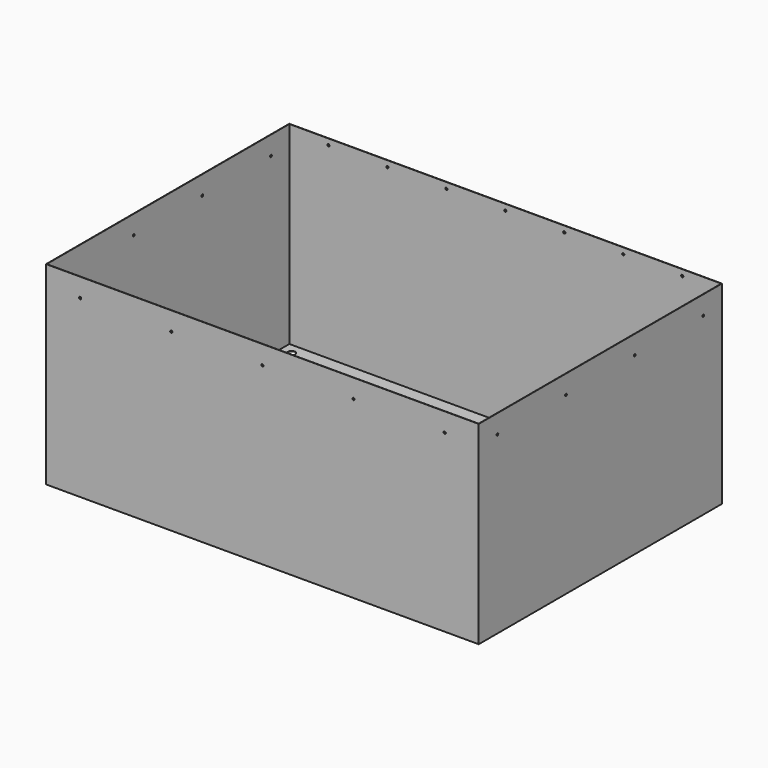
from build123d import *

# Parameters (mm, degrees)
F1_DEPTH  = 459.486
F2_T      = -0.762
F5_D      = 5.2197
F5_DEPTH  = 0.762
F5_TIP    = 1.5681560866
F6_D      = 5.2197
F8_D      = 49.022
F10_D     = 17.4625
F13_D     = 5.2197
F13_DEPTH = 0.762
F13_TIP   = 1.5681560866


# Not quite as in the source:
# - a length typed as a fraction of an inch, garbled in the dataset ("3 / 203.2 mm" for 3/8 in), is restored


with BuildPart() as f1:
    # F0 (on Top) → F1 (new body)
    with BuildSketch(Plane.XY):
        Polygon((0, 360.045), (-512.445, 360.045), (-512.445, -360.045), (0, -360.045), (0, 0), align=None)
        Polygon((512.445, 360.045), (0, 360.045), (0, 0), (0, -360.045), (512.445, -360.045), align=None)
    extrude(amount=F1_DEPTH)

    # F2
    f2_openings = [f1.faces().sort_by_distance(p)[0] for p in [
        (0, 0, 459.486),
    ]]
    offset(amount=F2_T, openings=f2_openings)

    # F5
    with Locations(Plane.XZ.offset(360.045)):
        with Locations((-431.8, 415.036), (-215.9, 415.036), (0, 415.036), (215.9, 415.036), (431.8, 415.036)):
            Hole(F5_D / 2, depth=F5_DEPTH)
            with Locations((0, 0, -(F5_DEPTH + F5_TIP / 2))):  # 118° drill point
                Cone(0, F5_D / 2, F5_TIP, mode=Mode.SUBTRACT)

    # F6 (through all)
    with Locations(Plane.YZ.offset(512.445)):
        with Locations((-304.8, 415.036), (-101.6, 415.036), (101.6, 415.036), (304.8, 415.036)):
            Hole(F6_D / 2)

    # F8 (through all)
    with Locations(Plane.XY.offset(0.762)):
        with Locations((-371.475, -193.675)):
            Hole(F8_D / 2)

    # F10 (through all)
    with Locations(Plane.XY.offset(0.762)):
        with Locations((-485.775, 333.375), (-485.775, -333.375), (485.775, -333.375), (485.775, 333.375)):
            Hole(F10_D / 2)

    # F13
    with Locations(Plane(origin=(0, 360.045, 0), x_dir=(-1, 0, 0), z_dir=(0, 1, 0))):
        with Locations((-419.1, 445.1985), (-279.4, 445.1985), (-139.7, 445.1985), (0, 445.1985), (139.7, 445.1985), (279.4, 445.1985), (419.1, 445.1985)):
            Hole(F13_D / 2, depth=F13_DEPTH)
            with Locations((0, 0, -(F13_DEPTH + F13_TIP / 2))):  # 118° drill point
                Cone(0, F13_D / 2, F13_TIP, mode=Mode.SUBTRACT)


solid = f1.part
